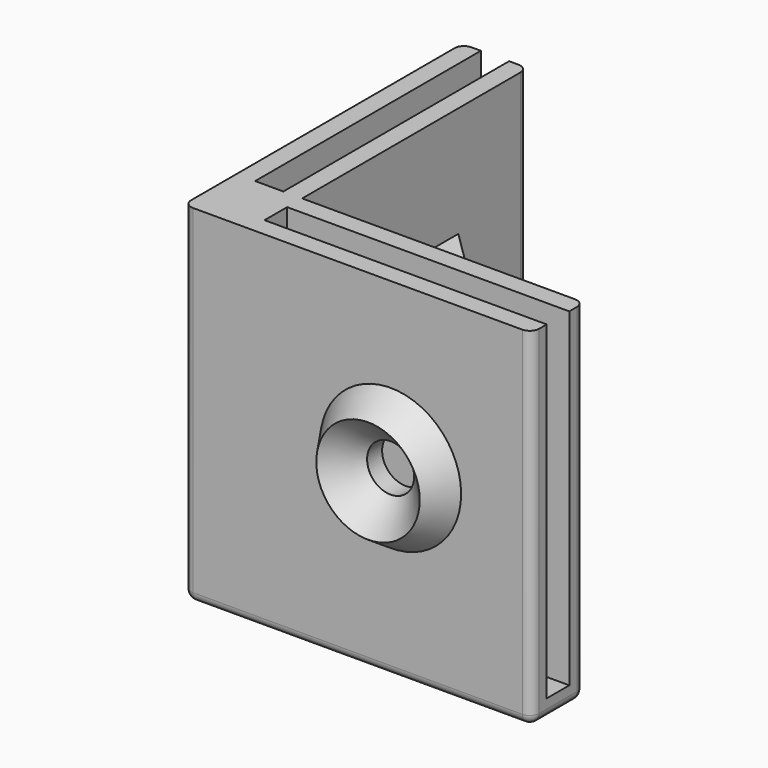
from build123d import *
from build123d import SkipClean  # not in build123d's __all__

# Parameters (mm, degrees)
F0_W          = 30
F0_H          = 37
F0_W_2        = 3
F0_H_2        = 35
F1_DEPTH      = 32
F2_DEPTH      = 25
F3_W          = 3
F3_H          = 35
F4_DEPTH      = 30
F5_W          = 11.5
F5_H          = 11.5
F6_DEPTH      = 2
F5_R          = 2.5
F7_DEPTH      = 25
F8_T4_DEPTH   = 21.8227903205
F8_T9_DEPTH   = 21.8227903205
F8_T14_DEPTH  = 21.8227903205
F8_T19_DEPTH  = 21.8227903205
F9_R          = 7.5
F9_R_2        = 2.5
F10_DEPTH     = 3
F11_SIZE      = 2.99999
F12_W         = 11.5
F12_H         = 11.5
F13_DEPTH     = 2
F14_T4_DEPTH  = 21.8227903205
F14_T9_DEPTH  = 21.8227903205
F14_T14_DEPTH = 21.8227903205
F14_T19_DEPTH = 21.8227903205
F12_R         = 2.5
F15_DEPTH     = 25
F16_R         = 7.5
F16_R_2       = 2.5
F17_DEPTH     = 3
F19_SIZE2     = 2.99999
F19_SIZE      = 1.99999
F19_2_SIZE2   = 2.99999
F19_2_SIZE    = 1.99999
F21_DEPTH     = 5
F22_R         = 1


# Not quite as in the source:
# - a fillet or chamfer that OpenCascade refuses, or shapes differently, is made with other operations: its cross-section is extruded or revolved along the edge and cut away or added
# - a fillet or chamfer is up to 0.001 mm smaller than in the source, because OpenCascade refuses the exact size
# - after a boolean that leaves OpenCascade's solid faulty, fix() repairs it


with BuildPart() as f1:
    # F0 (on Front) → F1 (new body)
    with BuildSketch(Plane.XZ):
        with Locations((3.5, 0)):
            Rectangle(F0_W, F0_H)
        Polygon((-18.5, -18.5), (-11.5, -18.5), (-11.5, 18.5), (-13.5, 18.5), (-13.5, -16.5), (-16.5, -16.5), (-16.5, 18.5), (-18.5, 18.5), align=None)
        with Locations((-15, 1)):
            Rectangle(F0_W_2, F0_H_2)
    extrude(amount=F1_DEPTH)

    # F0 (on Front) → F2 (cut)
    with BuildSketch(Plane.XZ):
        with Locations((3.5, 0)):
            Rectangle(F0_W, F0_H)
        with Locations((-15, 1)):
            Rectangle(F0_W_2, F0_H_2)
    extrude(amount=F2_DEPTH, mode=Mode.SUBTRACT)

    # F3 (on face) → F4 (cut)
    with BuildSketch(Plane.YZ.offset(18.5)):
        with Locations((-28.5, 1)):
            Rectangle(F3_W, F3_H)
    extrude(amount=-F4_DEPTH, mode=Mode.SUBTRACT)

    # F5 (on face) → F6 (join)
    with BuildSketch(Plane(origin=(0, -25, 0), x_dir=(-1, 0, 0), z_dir=(0, 1, 0))):
        with Locations((-3.5, 1)):
            Rectangle(F5_W, F5_H)
        Polygon((-8.1188021535, 1), (-5.8094010768, 5), (-1.1905989232, 5), (1.1188021535, 1), (-1.1905989232, -3), (-5.8094010768, -3), align=None, mode=Mode.SUBTRACT)
    extrude(amount=F6_DEPTH)

    # F5 (on face) → F7 (cut)
    with BuildSketch(Plane(origin=(0, -25, 0), x_dir=(-1, 0, 0), z_dir=(0, 1, 0))):
        with Locations((-3.5, 1)):
            Circle(F5_R)
    extrude(amount=-F7_DEPTH, mode=Mode.SUBTRACT)

    # F8: chamfer of 1.5 x 2 on 4 edges, made by hand


with BuildPart() as f8_tool2:
    # F8_s3 → F8_t4 (new body)
    with BuildSketch(Plane.XY.offset(11.9113951602)):
        Polygon((9.25, -25), (7.75, -23), (9.25, -23), align=None)
    extrude(amount=-F8_T4_DEPTH)

    split(bisect_by=Plane.XZ.offset(25), keep=Keep.BOTTOM)


with BuildPart() as f1_1:
    add(f1.part, clean=False)

    # F8_t1: cut F8_tool2
    add(f8_tool2.part, mode=Mode.SUBTRACT)


with BuildPart() as f8_tool7:
    # F8_s8 → F8_t9 (new body)
    with BuildSketch(Plane.YZ.offset(-7.4113951602)):
        Polygon((-25, 6.75), (-23, 5.25), (-23, 6.75), align=None)
    extrude(amount=F8_T9_DEPTH)

    split(bisect_by=Plane.XZ.offset(25), keep=Keep.BOTTOM)


with BuildPart() as f1_2:
    add(f1_1.part, clean=False)

    # F8_t6: cut F8_tool7
    add(f8_tool7.part, mode=Mode.SUBTRACT)


with BuildPart() as f8_tool12:
    # F8_s13 → F8_t14 (new body)
    with BuildSketch(Plane.XY.offset(-9.9113951602)):
        Polygon((-2.25, -25), (-0.75, -23), (-2.25, -23), align=None)
    extrude(amount=F8_T14_DEPTH)

    split(bisect_by=Plane.XZ.offset(25), keep=Keep.BOTTOM)


with BuildPart() as f1_3:
    add(f1_2.part, clean=False)

    # F8_t11: cut F8_tool12
    add(f8_tool12.part, mode=Mode.SUBTRACT)


with BuildPart() as f8_tool17:
    # F8_s18 → F8_t19 (new body)
    with BuildSketch(Plane.YZ.offset(14.4113951602)):
        Polygon((-25, -4.75), (-23, -3.25), (-23, -4.75), align=None)
    extrude(amount=-F8_T19_DEPTH)

    split(bisect_by=Plane.XZ.offset(25), keep=Keep.BOTTOM)


with BuildPart() as f1_4:
    add(f1_3.part, clean=False)

    # F8_t16: cut F8_tool17
    add(f8_tool17.part, mode=Mode.SUBTRACT)

    # F9 (on face) → F10 (join)
    with BuildSketch(Plane.XZ.offset(32)):
        with Locations((3.5, 1)):
            Circle(F9_R)
        with Locations((3.5, 1)):
            Circle(F9_R_2, mode=Mode.SUBTRACT)
    with SkipClean():  # cleaning this boolean's faces spoils the solid; the shape is the same uncleaned
        extrude(amount=F10_DEPTH)

    # F11 (size 3 in the source; OpenCascade refuses exactly that, so slightly less here)
    f11_edges = [f1_4.edges().sort_by_distance(p)[0] for p in [
        (1, -35, 1),
    ]]
    chamfer(f11_edges, length=F11_SIZE)

    # F12 (on face) → F13 (join)
    with BuildSketch(Plane.YZ.offset(-11.5)):
        with Locations((-10, 1)):
            Rectangle(F12_W, F12_H)
        Polygon((-10, 5.6188021535), (-6, 3.3094010768), (-6, -1.3094010768), (-10, -3.6188021535), (-14, -1.3094010768), (-14, 3.3094010768), align=None, mode=Mode.SUBTRACT)
    extrude(amount=F13_DEPTH)

    add(f1_4.part.fix(), mode=Mode.REPLACE)

    # F14: chamfer of 1.5 x 2 on 4 edges, made by hand


with BuildPart() as f14_tool2:
    # F14_s3 → F14_t4 (new body)
    with BuildSketch(Plane.XY.offset(-9.9113951602)):
        Polygon((-11.5, -4.25), (-9.5, -5.75), (-9.5, -4.25), align=None)
    extrude(amount=F14_T4_DEPTH)

    split(bisect_by=Plane.YZ.offset(-11.5), keep=Keep.TOP)


with BuildPart() as f1_5:
    add(f1_4.part, clean=False)

    # F14_t1: cut F14_tool2
    add(f14_tool2.part, mode=Mode.SUBTRACT)


with BuildPart() as f14_tool7:
    # F14_s8 → F14_t9 (new body)
    with BuildSketch(Plane.XZ.offset(20.9113951602)):
        Polygon((-11.5, -4.75), (-9.5, -3.25), (-9.5, -4.75), align=None)
    extrude(amount=-F14_T9_DEPTH)

    split(bisect_by=Plane.YZ.offset(-11.5), keep=Keep.TOP)


with BuildPart() as f1_6:
    add(f1_5.part, clean=False)

    # F14_t6: cut F14_tool7
    add(f14_tool7.part, mode=Mode.SUBTRACT)


with BuildPart() as f14_tool12:
    # F14_s13 → F14_t14 (new body)
    with BuildSketch(Plane.XY.offset(11.9113951602)):
        Polygon((-11.5, -15.75), (-9.5, -14.25), (-9.5, -15.75), align=None)
    extrude(amount=-F14_T14_DEPTH)

    split(bisect_by=Plane.YZ.offset(-11.5), keep=Keep.TOP)


with BuildPart() as f1_7:
    add(f1_6.part, clean=False)

    # F14_t11: cut F14_tool12
    add(f14_tool12.part, mode=Mode.SUBTRACT)


with BuildPart() as f14_tool17:
    # F14_s18 → F14_t19 (new body)
    with BuildSketch(Plane.XZ.offset(-0.9113951602)):
        Polygon((-11.5, 6.75), (-9.5, 5.25), (-9.5, 6.75), align=None)
    extrude(amount=F14_T19_DEPTH)

    split(bisect_by=Plane.YZ.offset(-11.5), keep=Keep.TOP)


with BuildPart() as f1_8:
    add(f1_7.part, clean=False)

    # F14_t16: cut F14_tool17
    add(f14_tool17.part, mode=Mode.SUBTRACT)

    # F12 (on face) → F15 (cut)
    with BuildSketch(Plane.YZ.offset(-11.5)):
        with Locations((-10, 1)):
            Circle(F12_R)
    extrude(amount=-F15_DEPTH, mode=Mode.SUBTRACT)

    # F16 (on face) → F17 (join)
    with BuildSketch(Plane(origin=(-18.5, 0, 0), x_dir=(0, -1, 0), z_dir=(-1, 0, 0))):
        with Locations((10, 1)):
            Circle(F16_R)
        with Locations((10, 1)):
            Circle(F16_R_2, mode=Mode.SUBTRACT)
    extrude(amount=F17_DEPTH)

    # F18: chamfer of 3 on 1 edges, made by hand

    # F18_s1 → F18_t2 (revolve, cut)
    with BuildSketch(Plane.XY.offset(1)):
        Polygon((-18.5, -12.5), (-21.5, -15.5), (-21.5, -12.5), align=None)
    revolve(axis=Axis((-21.5, -10, 1), (-1, 0, 0)), mode=Mode.SUBTRACT)

    # F19 (size 2 and 3 in the source; OpenCascade refuses exactly that, so slightly less here)
    f19_edges = [f1_8.edges().sort_by_distance(p)[0] for p in [
        (-21.5, -2.5, 1),
    ]]
    f19_side = f1_8.faces().sort_by_distance((-21.5, -2.712132, 1))[0]
    chamfer(f19_edges, length=F19_SIZE, length2=F19_SIZE2, reference=f19_side)

    # F19#2 (size 2 and 3 in the source; OpenCascade refuses exactly that, so slightly less here)
    f19_2_edges = [f1_8.edges().sort_by_distance(p)[0] for p in [
        (-4, -35, 1),
    ]]
    f19_2_side = f1_8.faces().sort_by_distance((-2.212122, -35, 1))[0]
    chamfer(f19_2_edges, length=F19_2_SIZE, length2=F19_2_SIZE2, reference=f19_2_side)

    # F20 (on face) → F21 (join)
    with BuildSketch(Plane(origin=(0, 0, 0), x_dir=(-1, 0, 0), z_dir=(0, 1, 0))):
        Polygon((11.5, -4.75), (11.5, -18.5), (18.5, -18.5), (18.5, 18.5), (16.5, 18.5), (16.5, -16.5), (13.5, -16.5), (13.5, 18.5), (11.5, 18.5), (11.5, 6.75), align=None)
    extrude(amount=F21_DEPTH)

    # F22
    f22_edges = [f1_8.edges().sort_by_distance(p)[0] for p in [
        (-11.5, 5, 0),
        (-18.5, 5, 0),
        (-11.5, -10, -18.5),
        (3.5, -25, -18.5),
        (0, -32, -18.5),
        (18.5, -32, 0),
        (18.5, -25, 0),
        (-15, 5, -18.5),
        (-18.5, -13.5, -18.5),
        (18.5, -28.5, -18.5),
        (-18.5, -32, 0),
    ]]
    fillet(f22_edges, radius=F22_R)


solid = f1_8.part
